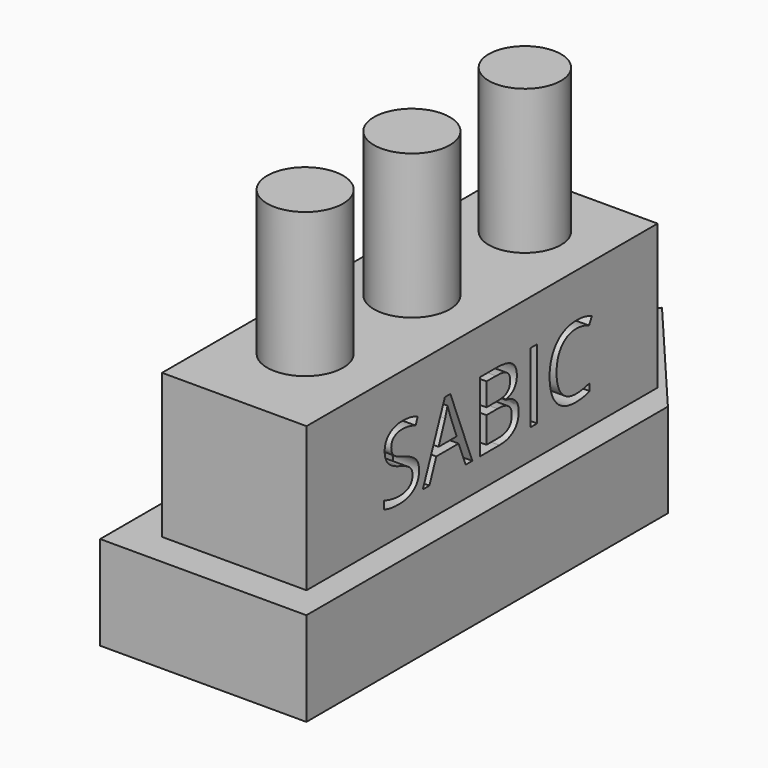
from build123d import *

# Parameters (mm, degrees)
F1_DEPTH     = 16.51
F2_W         = 25.4
F2_H         = 77.1319456398
F3_DEPTH     = 25.4
F4_TEXT_SIZE = 17.1883988919
F5_DEPTH     = 4.572
F6_R         = 6.35
F6_R_2       = 6.6705238581
F6_R_3       = 6.6705246024
F7_DEPTH     = 25.4


# Not quite as in the source:
# - Text() gives the source's letters only with a copy of the font that has no kerning and outlines rounded to 1/6400 em; it was checked with that copy


with BuildPart() as f1:
    # F0 (on Top) → F1 (new body)
    with BuildSketch(Plane.XY):
        Polygon((20.0875289738, 34.0563312852), (1.0928409174, 56.5046072006), (-16.1755010486, 34.0557545424), (-16.1755010486, -45.3786328435), (20.0875289738, -45.3786328435), align=None)
    extrude(amount=F1_DEPTH)

    # F2 (on face) → F3 (join)
    with BuildSketch(Plane.XY.offset(16.51)):
        with Locations((2.7707006454, -1.0073203593)):
            Rectangle(F2_W, F2_H)
    extrude(amount=F3_DEPTH)

    # F4 (on face) → F5 (cut)
    with BuildSketch(Plane.YZ.offset(15.4707006454)):
        with Locations((-23.4561692923, 21.7293333262)):
            Text('SABIC', F4_TEXT_SIZE, font='Open Sans', text_align=(TextAlign.LEFT, TextAlign.BOTTOM))
    extrude(amount=-F5_DEPTH, mode=Mode.SUBTRACT)

    # F6 (on face) → F7 (join)
    with BuildSketch(Plane.XY.offset(41.91)):
        with Locations((2.7341560926, 24.3195872754)):
            Circle(F6_R)
        with Locations((2.4463504087, -0.1439028856)):
            Circle(F6_R_2)
        with Locations((1.8707360141, -22.8805579245)):
            Circle(F6_R_3)
    extrude(amount=F7_DEPTH)


solid = f1.part
